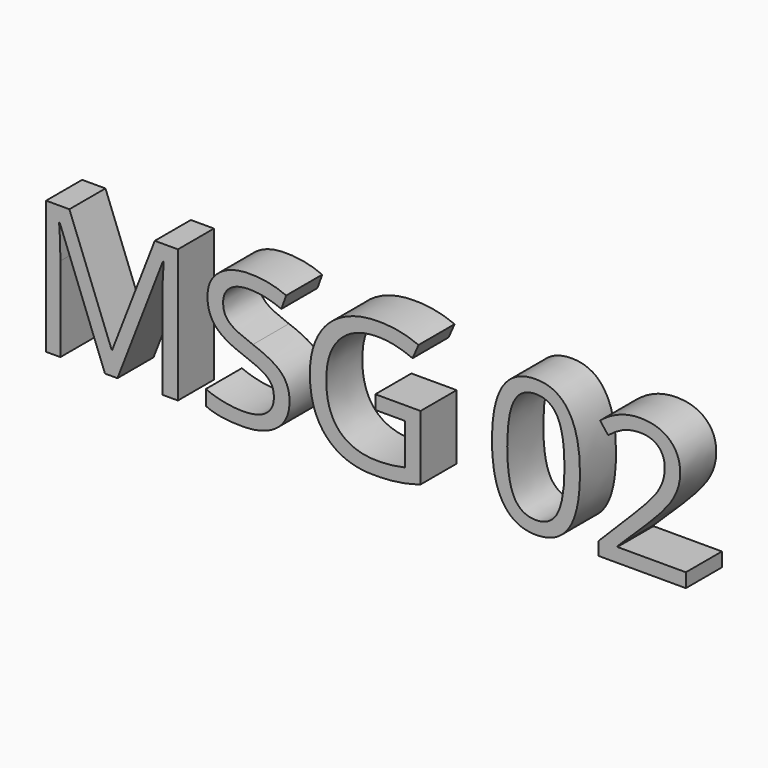
from build123d import *

# Parameters (mm, degrees)
F0_TEXT_SIZE = 105.0444475065
F1_DEPTH     = 25.4


# Not quite as in the source:
# - Text() gives the source's letters only with a copy of the font that has no kerning and outlines rounded to 1/6400 em; it was checked with that copy


with BuildPart() as f1:
    # F0 (on Front) → F1 (new body)
    with BuildSketch(Plane.XZ):
        with Locations((-127.5120228529, -43.598625809)):
            Text('MSG 02', F0_TEXT_SIZE, font='Open Sans', text_align=(TextAlign.LEFT, TextAlign.BOTTOM))
    extrude(amount=F1_DEPTH)


solid = f1.part
